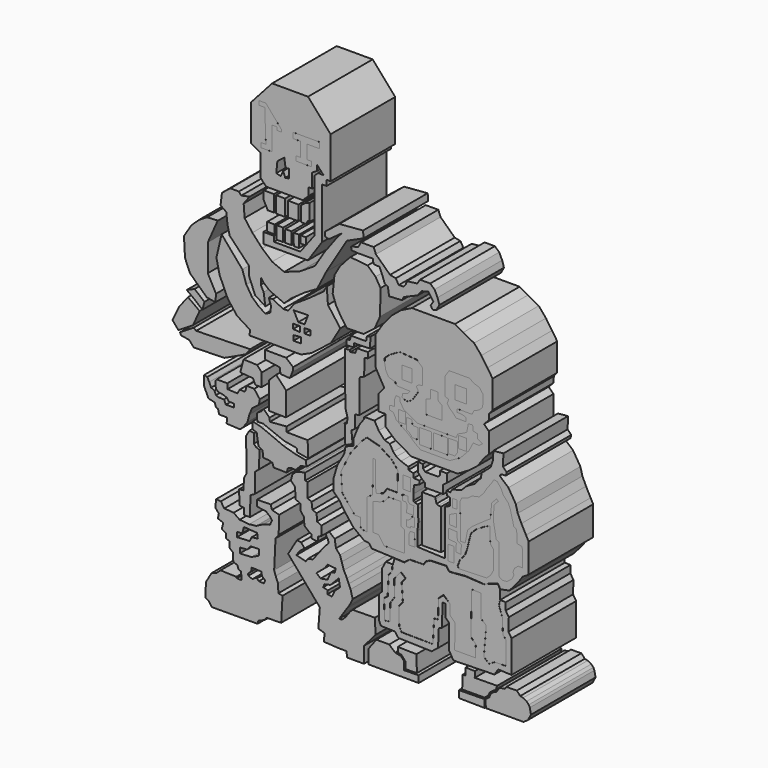
from build123d import *

# Parameters (mm, degrees)
F1_DEPTH      = 12.7
F1_DEPTH_BACK = 12.7
F0_W          = 2.3451782763
F0_H          = 2.7289353311
F3_DEPTH      = 12.7
F3_DEPTH_BACK = 12.7
F2_W          = 3.1842617318
F2_H          = 4.0236283094
F2_W_2        = 3.6299433559
F2_H_2        = 4.2267246172
F2_W_3        = 1.8677245826
F2_H_3        = 4.6415366232
F2_W_4        = 1.5032105148
F2_H_4        = 2.5777257979
F2_W_5        = 3.182772547
F2_H_5        = 4.0222080424
F2_W_6        = 3.6285351962
F2_H_6        = 4.2254780419
F2_W_7        = 2.2105854005
F2_H_7        = 3.4294971265
F2_W_8        = 1.8693469465
F2_H_8        = 4.6432167292
F2_W_9        = 1.5042312443
F2_H_9        = 2.5786831975
F2_W_10       = 3.7808120251
F2_H_10       = 4.7481860965
F2_W_11       = 4.3708886951
F2_H_11       = 4.6935402788
F2_W_12       = 2.4654623121
F2_H_12       = 3.6471767817
F2_W_13       = 2.2135460749
F2_H_13       = 3.4322766587
F2_W_14       = 3.7859473377
F2_H_14       = 4.7525740229
F2_W_15       = 4.3766628951
F2_H_15       = 4.6988725662
F2_W_16       = 2.4702642113
F2_H_16       = 3.651695326


# Not quite as in the source:
# - a feature names something its author has since deleted; it is built from what else it names


with BuildPart() as f1:
    # F0 (on Front) → F1 (new body, two sides)
    with BuildSketch(Plane.XZ) as f1_sk:
        Polygon((-9.5938611776, 66.9106543064), (-16.6862662882, 74.9939456582), (-27.994306758, 74.9939456582), (-34.6385799348, 67.5830319524), (-34.6385799348, 56.2110990286), (-31.6603220999, 54.5591711998), (-31.6603220999, 47.6847961545), (-29.7909770161, 45.815449208), (-18.3336883783, 45.815449208), (-16.5246427059, 47.5641936064), (-16.5246427059, 49.9762557447), (-15.3789138421, 49.9762557447), (-15.3789138421, 54.4385686517), (-13.9103056863, 55.3104877472), (-13.9103056863, 57.1270510554), (-11.8339713663, 54.8590533435), (-13.5205361214, 54.8850011104), (-14.5949935541, 53.9049506187), (-14.5949935541, 37.3129360378), (-17.3938885863, 33.6037576199), (-19.1130582243, 31.3254632056), (-27.4183992296, 31.3254632056), (-27.4183992296, 32.9865328968), (-30.7405348867, 32.9865328968), (-30.7405348867, 29.6643972397), (-16.7492311448, 29.6643972397), (-12.3410113156, 36.1170060933), (-12.3410113156, 52.1527044475), (-10.8716050163, 52.1527044475), (-10.8716050163, 53.877659142), (-9.5938611776, 53.877659142), align=None)
        Polygon((-26.3316370547, 54.0427602828), (-24.165680632, 55.7010732591), (-23.7595625222, 52.9597811401), (-22.728053189, 53.1125976231), (-22.728053189, 50.3538660705), (-23.861091584, 50.2184927464), (-24.5041102171, 51.8768019974), (-25.3163445741, 50.184648484), (-26.6700685024, 50.5569241941), align=None, mode=Mode.SUBTRACT)
        Polygon((-31.4840041101, 57.4934072793), (-29.9422182143, 57.4934072793), (-30.3007718176, 67.6046609879), (-32.0935472846, 67.6046609879), (-32.0935472846, 68.8936337829), (-29.9574602395, 68.8936337829), (-24.9686259777, 63.0946457386), (-24.9686259777, 62.4657310545), (-26.4403745532, 62.4657310545), (-26.5174116939, 63.4554550052), (-28.077730909, 63.4554550052), (-28.077730909, 56.0591891408), (-31.4840041101, 56.0591891408), align=None, mode=Mode.SUBTRACT)
        Polygon((-21.3707555085, 61.8773698807), (-21.3707555085, 63.4141266346), (-21.3707555085, 63.6133402586), (-13.1177809089, 63.6133402586), (-13.1177809089, 61.763536185), (-16.9881414622, 61.763536185), (-16.9881414622, 57.4662983418), (-15.6221324578, 57.4662983418), (-15.6221324578, 55.9295378625), (-20.4316228628, 55.9295378625), (-20.4316228628, 57.4093796313), (-19.0371554345, 57.4093796313), (-19.0371554345, 61.8773698807), align=None, mode=Mode.SUBTRACT)
    extrude(amount=F1_DEPTH)
    extrude(f1_sk.sketch, amount=-F1_DEPTH_BACK)


with BuildPart() as f1b:
    # F0 (on Front) → F1, piece 2 (new body, two sides)
    with BuildSketch(Plane.XZ) as f1_2_sk:
        Polygon((-30.6372623891, 44.5467084646), (-30.6372623891, 44.2908704281), (-30.6372623891, 41.903052479), (-29.358074069, 39.4299551845), (-27.3966528475, 39.4299551845), (-27.3966528475, 44.5467084646), align=None)
    extrude(amount=F1_DEPTH)
    extrude(f1_2_sk.sketch, amount=-F1_DEPTH_BACK)


with BuildPart() as f1c:
    # F0 (on Front) → F1, piece 3 (new body, two sides)
    with BuildSketch(Plane.XZ) as f1_3_sk:
        Polygon((-23.9142030478, 44.4402880967), (-26.7252419144, 44.472232461), (-26.7252419144, 39.3612533808), (-23.9142030478, 39.3612533808), align=None)
    extrude(amount=F1_DEPTH)
    extrude(f1_3_sk.sketch, amount=-F1_DEPTH_BACK)


with BuildPart() as f1d:
    # F0 (on Front) → F1, piece 4 (new body, two sides)
    with BuildSketch(Plane.XZ) as f1_4_sk:
        Polygon((-19.6976456791, 44.1527962685), (-22.9558944702, 44.1847406328), (-22.9558944702, 39.5529158413), (-19.6976456791, 39.5529158413), align=None)
    extrude(amount=F1_DEPTH)
    extrude(f1_4_sk.sketch, amount=-F1_DEPTH_BACK)


with BuildPart() as f1e:
    # F0 (on Front) → F1, piece 5 (new body, two sides)
    with BuildSketch(Plane.XZ) as f1_5_sk:
        Polygon((-17.4935366958, 45.2708229423), (-18.8671126962, 44.2805700004), (-18.8671126962, 39.5529158413), (-17.1741005033, 39.5529158413), (-16.8227199465, 40.5431687832), (-16.1519050598, 40.5431687832), (-16.1519050598, 45.7819215953), align=None)
    extrude(amount=F1_DEPTH)
    extrude(f1_5_sk.sketch, amount=-F1_DEPTH_BACK)


with BuildPart() as f1f:
    # F0 (on Front) → F1, piece 6 (new body, two sides)
    with BuildSketch(Plane.XZ) as f1_6_sk:
        Polygon((-19.0333388746, 33.6037576199), (-17.3938885863, 33.6037576199), (-17.3938885863, 35.8636565506), (-19.0333388746, 35.8636565506), (-19.0333388746, 35.5651788414), align=None)
    extrude(amount=F1_DEPTH)
    extrude(f1_6_sk.sketch, amount=-F1_DEPTH_BACK)


with BuildPart() as f1g:
    # F0 (on Front) → F1, piece 7 (new body, two sides)
    with BuildSketch(Plane.XZ) as f1_7_sk:
        Polygon((-21.2505981326, 35.8636565506), (-21.1653206497, 32.1540087461), (-19.5450149477, 32.1540087461), (-19.5450149477, 35.8636565506), align=None)
    extrude(amount=F1_DEPTH)
    extrude(f1_7_sk.sketch, amount=-F1_DEPTH_BACK)


with BuildPart() as f1h:
    # F0 (on Front) → F1, piece 8 (new body, two sides)
    with BuildSketch(Plane.XZ) as f1_8_sk:
        Polygon((-23.8516163081, 36.0342152417), (-23.8942559808, 32.1966484189), (-21.8475535512, 32.1966484189), (-21.8475535512, 36.0342152417), align=None)
    extrude(amount=F1_DEPTH)
    extrude(f1_8_sk.sketch, amount=-F1_DEPTH_BACK)


with BuildPart() as f1i:
    # F0 (on Front) → F1, piece 9 (new body, two sides)
    with BuildSketch(Plane.XZ) as f1_9_sk:
        Polygon((-26.5379119664, 36.2047739327), (-26.623191312, 32.1966484189), (-24.5338492095, 32.1966484189), (-24.5338492095, 36.2047739327), align=None)
    extrude(amount=F1_DEPTH)
    extrude(f1_9_sk.sketch, amount=-F1_DEPTH_BACK)


with BuildPart() as f1j:
    # F0 (on Front) → F1, piece 10 (new body, two sides)
    with BuildSketch(Plane.XZ) as f1_10_sk:
        with Locations((-28.3500943333, 34.8403062671)):
            Rectangle(F0_W, F0_H)
    extrude(amount=F1_DEPTH)
    extrude(f1_10_sk.sketch, amount=-F1_DEPTH_BACK)


with BuildPart() as f1k:
    # F0 (on Front) → F1, piece 11 (new body, two sides)
    with BuildSketch(Plane.XZ) as f1_11_sk:
        Polygon((-36.9369212724, 38.8479313689), (-35.0333526731, 41.3705967367), (-37.6954227686, 40.775667876), (-38.418225944, 41.6791699827), (-41.128732264, 41.6791699827), (-43.7488853931, 39.6011136472), (-44.2006364465, 35.9871052206), (-42.3936359584, 34.7222052515), (-42.0322343707, 31.4695984125), (-41.3094311953, 28.488041833), (-35.2559685707, 22.1635270864), (-35.2559685707, 19.3626713008), (-33.3586148918, 14.6644618362), (-30.1060080528, 12.5864073634), (-30.6481085718, 16.3811147213), (-31.5516106784, 18.097769469), (-31.42894949, 20.0820728757), (-30.6238532066, 18.9463123679), (-28.6898408085, 17.3346363008), (-24.1771470755, 15.4006257653), (-21.9745226204, 17.4420811236), (-17.7304428071, 20.4505436122), (-13.8624189422, 22.7068904787), (-10.961400345, 28.4014809877), (-4.491341766, 39.0913411975), (0.7715018001, 41.4606525215), (0.5989942583, 43.5738749802), (-6.8465704098, 42.9660752416), (-11.3291051239, 39.3952429295), (-11.3291051239, 38.0276888609), (-10.1135037839, 37.7237871289), (-6.0868188739, 40.610846132), (-7.7582728118, 38.7114658952), (-11.4810559899, 33.6971059442), (-14.5200621337, 28.8346949965), (-19.1545449197, 25.8716642857), (-24.1689067334, 24.0482613444), (-27.9676634818, 25.6437398493), (-31.0826450586, 28.3028688282), (-34.1976247728, 31.6457748413), (-36.6288311779, 34.9127091467), align=None)
    extrude(amount=F1_DEPTH)
    extrude(f1_11_sk.sketch, amount=-F1_DEPTH_BACK)


with BuildPart() as f1l:
    # F0 (on Front) → F1, piece 12 (new body, two sides)
    with BuildSketch(Plane.XZ) as f1_12_sk:
        Polygon((-0.9377481183, 38.5080315173), (-3.0890780035, 37.9343405366), (-3.1607891433, 37.7909205854), (-2.9456561897, 36.9303897023), (-1.2245918624, 36.7869660258), (3.723466536, 36.7869660258), (3.8668890484, 35.3527478874), (5.8030853979, 35.2093242109), (6.663617678, 33.2014150918), (7.3807276785, 31.1935078353), (8.3846813068, 30.6198205799), (8.8149476796, 28.0382242054), (12.8307631239, 28.2533578575), (13.4044513106, 29.3290223926), (15.0538031012, 30.0461333245), (17.7788212895, 31.1935078353), (18.9979076385, 32.7711515129), (21.1492385715, 33.3448387682), (22.7268803865, 31.0500860214), (21.8663476408, 29.8309996724), (22.4400348961, 28.7553351372), (23.6591231078, 29.0421787649), (24.5913658291, 30.7632423937), (24.0176785737, 32.6277278364), (23.0854358524, 34.5639251173), (21.7229258269, 35.7830114663), (18.4959303588, 35.7830114663), (17.6354013383, 34.4205051661), (14.4084058702, 34.0619497001), (13.978138566, 32.9145714641), (13.4044513106, 32.1974642575), (11.8268085644, 32.1257524192), (10.894565843, 33.7033942342), (9.1017913073, 34.0619497001), (4.6557090245, 38.2928960025), (3.938599024, 40.0856733322), (0, 40.0856733322), align=None)
    extrude(amount=F1_DEPTH)
    extrude(f1_12_sk.sketch, amount=-F1_DEPTH_BACK)


with BuildPart() as f1m:
    # F0 (on Front) → F1, piece 13 (new body, two sides)
    with BuildSketch(Plane.XZ) as f1_13_sk:
        Polygon((2.0290226676, 34.3684926629), (-3.3819169391, 34.9032784963), (-5.0103398971, 33.2014150918), (-6.7701800726, 31.1195589602), (-8.394648321, 28.276739642), (-8.936136961, 22.9972191155), (-7.8531587496, 20.0190264732), (-6.0933185741, 17.1085204929), (-4.4688507915, 14.8748783395), (0.8106696187, 15.0102507323), (4.1949781589, 17.5823252648), (5.9548197314, 21.508121863), (6.0901925899, 29.4274035841), (4.5334086753, 32.0671647787), align=None)
    extrude(amount=F1_DEPTH)
    extrude(f1_13_sk.sketch, amount=-F1_DEPTH_BACK)


with BuildPart() as f1n:
    # F0 (on Front) → F1, piece 14 (new body, two sides)
    with BuildSketch(Plane.XZ) as f1_14_sk:
        Polygon((-37.35839203, 20.4856079072), (-43.8636057079, 28.0750244856), (-45.4980805516, 21.0728552192), (-44.4747321308, 16.553055495), (-41.9163554907, 10.8393486589), (-39.0168614686, 7.087062113), (-34.9234566092, 4.5286854729), (-35.0940153003, 2.908379538), (-18.8909620047, 2.908379538), (-15.6503524631, 4.3581272475), (-9.5305331051, 9.1014830396), (-6.5489741974, 14.1610940918), (-10.4340352118, 19.4014050066), (-10.7954340056, 24.3706665933), (-11.7892883718, 22.6540118456), (-16.6681967676, 19.1303547472), (-20.8243075758, 16.4198484272), (-22.9927096516, 13.7093439698), (-24.5286636055, 13.7093439698), (-27.7812685817, 15.335646458), (-29.0461741388, 15.335646458), (-28.323372826, 13.2575919852), (-28.5944230855, 11.2698879093), (-30.1303770393, 10.5470865965), (-32.2987772524, 11.9926892221), (-34.2864841223, 13.7996925041), (-36.0934883356, 16.6908986866), align=None)
        Polygon((-21.2671738118, 5.9554395266), (-21.2671738118, 7.5206770562), (-18.9672354609, 7.7123385854), (-18.9672354609, 5.9554395266), align=None, mode=Mode.SUBTRACT)
        Polygon((-21.3949494064, 9.1498009861), (-21.3949494064, 10.6511516497), (-19.1588960588, 10.6511516497), (-19.1588960588, 8.9900828898), align=None, mode=Mode.SUBTRACT)
        Polygon((-19.7437535971, 11.6068609059), (-20.9376644343, 13.9094004408), (-21.1935024709, 14.4210755825), (-16.6737027466, 14.506354928), (-17.7823323756, 11.6068609059), align=None, mode=Mode.SUBTRACT)
        Polygon((-17.8172644228, 9.0539706871), (-17.8172644228, 10.5872638524), (-15.9006472677, 10.6511516497), (-15.9006472677, 9.0539706871), align=None, mode=Mode.SUBTRACT)
    extrude(amount=F1_DEPTH)
    extrude(f1_14_sk.sketch, amount=-F1_DEPTH_BACK)


with BuildPart() as f1o:
    # F0 (on Front) → F1, piece 15 (new body, two sides)
    with BuildSketch(Plane.XZ) as f1_15_sk:
        Polygon((-48.2119210064, 24.4022365659), (-45.1531931758, 31.3246250153), (-44.9922047555, 31.4856097102), (-48.4028458595, 31.2973856926), (-50.9676299989, 29.741641134), (-53.3509030938, 27.4967011064), (-55.6977577507, 23.7582940608), (-55.3757883608, 17.8018212318), (-53.8464225829, 14.0991490334), (-50.7876947522, 11.2014058977), (-48.5338903964, 9.1085908934), (-45.7971356809, 8.6256340146), (-45.636150986, 11.0404202715), (-48.2119210064, 15.8699918538), align=None)
    extrude(amount=F1_DEPTH)
    extrude(f1_15_sk.sketch, amount=-F1_DEPTH_BACK)


with BuildPart() as f1p:
    # F0 (on Front) → F1, piece 16 (new body, two sides)
    with BuildSketch(Plane.XZ) as f1_16_sk:
        Polygon((-52.33906582, 10.1660164073), (-54.8434145749, 9.0845925733), (-52.5667332113, 7.4339979328), (-49.8916320503, 5.2142329514), (-49.2655448616, 7.6047494076), align=None)
    extrude(amount=F1_DEPTH)
    extrude(f1_16_sk.sketch, amount=-F1_DEPTH_BACK)


with BuildPart() as f1q:
    # F0 (on Front) → F1, piece 17 (new body, two sides)
    with BuildSketch(Plane.XZ) as f1_17_sk:
        Polygon((-50.790656358, 4.5965607278), (-54.4437915087, 7.2289654054), (-57.129919529, 3.7907224614), (-59.3325421214, -0.6682488602), (-57.4522539973, -2.8708733153), (-52.8321154416, 0), align=None)
    extrude(amount=F1_DEPTH)
    extrude(f1_17_sk.sketch, amount=-F1_DEPTH_BACK)


with BuildPart() as f1r:
    # F0 (on Front) → F1, piece 18 (new body, two sides)
    with BuildSketch(Plane.XZ) as f1_18_sk:
        Polygon((-52.617225796, -0.6145262741), (-56.9150298834, -3.3006537706), (-56.6464141011, -4.0527693927), (-54.0677346289, -4.4825496152), (-52.617225796, -6.094226148), (-43.0546104908, -5.8793355711), (-39.5626462996, -4.267659504), (-36.2318493426, -2.655983204), (-34.8887853324, -0.8294165018), (-51.8651083112, -1.2591967825), align=None)
    extrude(amount=F1_DEPTH)
    extrude(f1_18_sk.sketch, amount=-F1_DEPTH_BACK)


with BuildPart() as f1s:
    # F0 (on Front) → F1, piece 19 (new body, two sides)
    with BuildSketch(Plane.XZ) as f1_19_sk:
        Polygon((-23.6031040549, 0.4885619273), (-30.1950573921, 0.5392691819), (-30.1950573921, -2.1482193843), (-25.5299843848, -2.8074146248), (-25.3778602928, -4.5821708627), (-22.4875435233, -4.7850008123), (-21.524105221, -2.7567071375), (-21.3719829917, -1.3876094017), align=None)
    extrude(amount=F1_DEPTH)
    extrude(f1_19_sk.sketch, amount=-F1_DEPTH_BACK)


with BuildPart() as f1t:
    # F0 (on Front) → F1, piece 20 (new body, two sides)
    with BuildSketch(Plane.XZ) as f1_20_sk:
        Polygon((-36.8002168834, -4.3107029051), (-36.9612015784, -4.3107029051), (-38.0076095462, -8.2548540086), (-33.9829660952, -8.5768252611), (-33.2585312426, -10.1866824552), (-31.3267037272, -10.1866824552), (-31.2462095171, -6.0815461911), (-32.695081085, -4.4716885313), align=None)
    extrude(amount=F1_DEPTH)
    extrude(f1_20_sk.sketch, amount=-F1_DEPTH_BACK)


with BuildPart() as f1u:
    # F0 (on Front) → F1, piece 21 (new body, two sides)
    with BuildSketch(Plane.XZ) as f1_21_sk:
        Polygon((-28.9138779044, -7.434383966), (-29.0096011013, -7.434383966), (-29.0096011013, -15.9537047148), (-23.6491281539, -16.049426049), (-23.5534086823, -8.5830567405), (-26.7122555524, -5.2327625453), align=None)
    extrude(amount=F1_DEPTH)
    extrude(f1_21_sk.sketch, amount=-F1_DEPTH_BACK)


with BuildPart() as f1v:
    # F0 (on Front) → F1, piece 22 (new body, two sides)
    with BuildSketch(Plane.XZ) as f1_22_sk:
        Polygon((-5.1528443582, -11.6437776014), (-4.9752146006, -17.6448337734), (-2.6907407378, -16.5448998462), (-3.0455661472, -12.9111642018), (-1.8998369342, -12.1272439137), (-1.929987804, -8.1473439932), (-0.5732035497, -7.9362886027), (-0.42929349, 2.6036400814), (0.9762255359, 3.2425122336), (0.9992049308, 8.3681419492), (2.2052354179, 8.7299505249), (2.0846324041, 10.4183927178), (-1.2922529131, 10.3580914438), (-1.8349663587, 8.9108552784), (-3.40280612, 8.6394986138), (-3.5535597708, 9.21236258), (-5.0912485458, 8.9711565524), (-4.961182829, -7.0438971743), (-4.7858525068, -7.9941847362), (-4.2383526452, -9.9451867864), (-4.5139719732, -11.4521170035), align=None)
    extrude(amount=F1_DEPTH)
    extrude(f1_22_sk.sketch, amount=-F1_DEPTH_BACK)


with BuildPart() as f1w:
    # F0 (on Front) → F1, piece 23 (new body, two sides)
    with BuildSketch(Plane.XZ) as f1_23_sk:
        Polygon((-3.4961928613, 11.9555769488), (-4.6345340088, 11.6994502023), (-4.6345340088, 10.1626897231), (-2.32939329, 10.2765234187), (-2.2155591287, 11.4717818797), (2.7931416407, 11.6140749305), (2.9354346916, 14.9437226355), (1.7970931949, 14.6591365337), (1.5694251051, 13.2362106815), (-3.2685245387, 13.2362106815), align=None)
    extrude(amount=F1_DEPTH)
    extrude(f1_23_sk.sketch, amount=-F1_DEPTH_BACK)


with BuildPart() as f1x:
    # F0 (on Front) → F1, piece 24 (new body, two sides)
    with BuildSketch(Plane.XZ) as f1_24_sk:
        Polygon((-32.6734371483, -17.6987983286), (-32.6734371483, -19.6284465492), (-32.5862728059, -20.1711598784), (-30.7437889278, -20.1108586043), (-28.5126324743, -21.0153814405), (-24.2312233895, -22.7038245648), (-20.2513244003, -23.4274435788), (-20.1307218522, -24.5128702372), (-16.6332330555, -25.1158848405), (-16.8141368777, -20.1108586043), (-23.4473049641, -20.0505573303), (-23.4473049641, -18.4827186167), (-28.6935362965, -18.9048293978), (-28.8141407073, -17.8194008768), (-30.6231863797, -16.0103552043), (-31.3468053937, -16.8545767665), align=None)
    extrude(amount=F1_DEPTH)
    extrude(f1_24_sk.sketch, amount=-F1_DEPTH_BACK)


with BuildPart() as f1y:
    # F0 (on Front) → F1, piece 25 (new body, two sides)
    with BuildSketch(Plane.XZ) as f1_25_sk:
        Polygon((-31.2966257334, -21.257204935), (-34.0757220984, -20.5111056566), (-34.0757220984, -22.7471590042), (-32.8299216926, -23.1943689287), (-32.2868786752, -26.7720539123), (-30.9771914035, -27.6025887579), (-30.7855289429, -29.5192059129), (-28.9008561522, -29.6469796449), (-27.8467163444, -29.9983602017), (-27.5272801518, -31.1802737415), (-23.4384965152, -31.2441606075), (-23.023230955, -29.9025289714), (-21.7774286866, -29.4872615486), (-20.5955151469, -29.5830927789), (-19.7330377996, -28.6886710674), (-18.9983341843, -27.9220249504), (-17.1775482595, -27.6025887579), (-17.3692107201, -25.8776322007), (-20.946893841, -25.1543261111), (-24.3968050927, -24.1640750319), (-27.3995064199, -22.8863302618), align=None)
    extrude(amount=F1_DEPTH)
    extrude(f1_25_sk.sketch, amount=-F1_DEPTH_BACK)


with BuildPart() as f1z:
    # F0 (on Front) → F1, piece 26 (new body, two sides)
    with BuildSketch(Plane.XZ) as f1_26_sk:
        Polygon((-43.0968850851, -17.3945352435), (-44.8567271233, -17.3945352435), (-45.6112548709, -17.0357543975), (-46.1307689548, -15.951551497), (-47.1697971225, -15.4546266422), (-47.7570705116, -14.0993734822), (-48.344347626, -12.8796454519), (-49.3616610765, -12.6537699252), (-49.3616610765, -15.761744231), (-47.9702912271, -18.7482573092), (-45.9973849356, -19.1603135318), (-45.6689596176, -20.3727260232), (-44.9827052653, -20.6235628575), (-44.6536689997, -22.0648795366), (-42.1492792666, -22.0648795366), (-42.2846525908, -23.8247197121), (-38.0881093442, -24.0277796984), (-37.2081883252, -23.2832320035), (-35.7190929353, -21.2526451796), (-35.1099185646, -18.9513172954), (-34.2976860702, -16.9884171337), (-32.1317277849, -15.2962636203), (-31.8609811366, -13.6717958376), (-33.6208231747, -11.3704660907), (-35.9221510589, -11.3027794287), (-36.531329155, -13.1303062662), (-38.155797869, -13.0626205355), (-38.9003455639, -14.3486568704), (-42.0139059424, -14.2132854089), (-42.0815944672, -12.5888166949), (-45.3982166946, -12.5888166949), (-45.7513257861, -13.1409596652), (-45.6944070756, -15.1330558583), (-44.9921004474, -15.9054398537), (-43.3676317334, -16.1761846393), (-42.2846525908, -16.5823008865), (-41.6077896953, -17.4622200429), (-39.9833209813, -17.529906705), (-39.9156361818, -18.6128858477), (-42.5553955138, -18.6805725098), align=None)
    extrude(amount=F1_DEPTH)
    extrude(f1_26_sk.sketch, amount=-F1_DEPTH_BACK)


with BuildPart() as f1ba:
    # F0 (on Front) → F1, piece 27 (new body, two sides)
    with BuildSketch(Plane.XZ) as f1_27_sk:
        Polygon((-33.6043462157, -23.650649935), (-35.135909915, -23.435274139), (-36.1285246909, -25.1578874886), (-36.0905379057, -35.6804467738), (-36.8502885103, -37.1619611979), (-36.9642525911, -40.580842644), (-38.3318029344, -40.6948067248), (-38.2938161492, -45.1773405075), (-36.8882752955, -45.3292913735), (-36.8123017251, -47.3046451807), (-34.9509119987, -47.3426319659), (-34.7989611328, -41.1886461079), (-33.4396325052, -40.4247939587), (-33.4396325052, -34.3261547387), (-32.0843793452, -33.1516042352), (-31.9770611823, -27.7427956462), (-33.0539382994, -27.3120421916), (-33.7239988148, -26.6180541366), align=None)
    extrude(amount=F1_DEPTH)
    extrude(f1_27_sk.sketch, amount=-F1_DEPTH_BACK)


with BuildPart() as f1bb:
    # F0 (on Front) → F1, piece 28 (new body, two sides)
    with BuildSketch(Plane.XZ) as f1_28_sk:
        Polygon((-18.8277959824, -29.6179540455), (-20.5805432051, -30.192617327), (-21.6056704521, -31.1802737415), (-22.0880825073, -33.0267883837), (-20.76144889, -34.3534238636), (-20.6408444792, -37.7303063869), (-19.0127044916, -38.3936241269), (-19.0730057657, -40.3232723475), (-17.9272778332, -41.8308116496), (-17.860205844, -44.0748855472), (-16.3803622127, -45.3839786351), (-15.6404413283, -45.7823984325), (-15.5835244805, -46.9207391143), (-13.6483442038, -47.1484065056), (-13.5345105082, -45.7823984325), (-12.3961688951, -45.1563112438), (-12.510003522, -42.3673763871), (-13.8760125265, -41.6843704879), (-13.9898471534, -39.4076891243), (-15.29893931, -38.9523506165), (-15.5835244805, -36.7895029485), (-16.8357007205, -36.2203344703), (-16.8357007205, -31.7238867283), (-17.5756216049, -31.5531343222), (-17.6325384527, -29.3902866542), align=None)
    extrude(amount=F1_DEPTH)
    extrude(f1_28_sk.sketch, amount=-F1_DEPTH_BACK)


with BuildPart() as f1bc:
    # F0 (on Front) → F1, piece 29 (new body, two sides)
    with BuildSketch(Plane.XZ) as f1_29_sk:
        Polygon((-28.4168235958, -41.6801795363), (-32.7146276832, -41.7402908206), (-32.7146276832, -43.6743050814), (-29.9210548401, -44.0503619611), (-28.631715104, -45.1248139143), (-28.040766716, -45.9843724966), (-28.631715104, -47.3811589181), (-30.6731704623, -47.9183867574), (-32.9832397401, -49.100279808), (-35.1858660579, -49.3688955903), (-38.1943285465, -49.100279808), (-40.0746166706, -47.7572157979), (-43.0293567479, -47.5423261523), (-44.103808701, -45.9306500852), (-45.6080399454, -45.8232052624), (-45.8229295909, -48.2407212257), (-44.7484776378, -49.5300628245), (-45.0170896947, -50.9805716574), (-43.3516912162, -51.6252405941), (-43.7814742327, -53.4518063068), (-42.4921326339, -54.2039237916), (-42.4921326339, -55.6007102132), (-41.4176806808, -56.0842119157), (-41.3639582694, -57.9107776284), (-40.3432287276, -58.770339936), (-40.1820614934, -61.2953007221), (-38.8927198946, -61.9399696589), (-38.5166630149, -63.0144178867), (-37.7645455301, -63.2293075323), (-37.5496558845, -65.6468272209), (-39.0538871288, -65.5931010842), (-39.215054363, -65.2170479298), (-44.2112535238, -65.0558769703), (-45.5005951226, -66.237770021), (-47.0048263669, -66.7212754488), (-48.7776696682, -69.7233527899), (-48.9925593138, -74.1285979748), (-47.9181073606, -74.7732669115), (-46.8973815441, -76.1163309216), (-32.553460449, -76.0626122355), (-32.284848392, -75.0418826938), (-31.3178412616, -74.7195482254), (-30.2433911711, -74.2360427976), (-29.8136100173, -73.483929038), (-25.1397490501, -73.3764842153), (-24.7099678963, -65.7478794456), (-25.9993094951, -65.4792711139), (-26.1604785919, -62.7394169569), (-26.85886994, -60.9665736556), (-27.3423735052, -59.5160648227), (-26.9125942141, -50.5981221795), (-25.9455870837, -49.3087805808), (-25.7306974381, -43.6679162085), (-28.040766716, -43.0769659579), align=None)
        Polygon((-34.1644622386, -64.2259716988), (-35.4741513729, -63.714876771), (-35.5060957372, -63.0760043859), (-34.579731524, -62.2454695404), (-34.451957792, -61.0954985023), (-31.3534252346, -61.2232722342), (-31.1937071383, -62.3732432723), (-30.1395691931, -63.3315518498), (-30.5548347533, -64.2259716988), (-32.1839600801, -64.1620829701), (-32.7589437366, -63.5870993137), (-33.2380980253, -63.5870993137), align=None, mode=Mode.SUBTRACT)
        Polygon((-38.1465218961, -58.3931319416), (-38.1465218961, -56.7442439497), (-35.8651801944, -56.5861277282), (-34.8487384617, -55.3438141942), (-32.1156457067, -55.2308782935), (-32.0478826761, -57.0378787816), (-34.487336874, -58.2124330103), align=None, mode=Mode.SUBTRACT)
        Polygon((-39.0662886202, -54.2039237916), (-39.0662886202, -52.7116432786), (-37.3587757349, -52.5978058577), (-36.8465222418, -50.6626293063), (-32.6915755868, -50.9472116828), (-32.4639081955, -52.483972162), (-34.3990884721, -52.7116432786), (-35.0251756608, -53.963817656), align=None, mode=Mode.SUBTRACT)
    extrude(amount=F1_DEPTH)
    extrude(f1_29_sk.sketch, amount=-F1_DEPTH_BACK)


with BuildPart() as f1bd:
    # F0 (on Front) → F1, piece 30 (new body, two sides)
    with BuildSketch(Plane.XZ) as f1_30_sk:
        Polygon((-19.426131621, -51.6865924001), (-17.7577332582, -50.3934485057), (-18.8531130552, -49.0724369884), (-20.1647710055, -48.8816089928), (-22.9407288134, -53.5720214248), (-12.9855694249, -65.1544630527), (-13.4641826153, -71.1849927902), (-11.5497289225, -71.7593356967), (-11.6454521194, -74.2481201887), (-6.9550401531, -74.5352879167), (-4.6576941386, -74.5352879167), (-4.3705268763, -76.2583017349), (0.8942213608, -76.2583017349), (0.8942206623, -71.2807178497), (4.5316843316, -67.0689195395), (4.3402379379, -62.3785071075), (-2.7432409115, -62.474232167), (-3.6047447938, -63.4314566851), (-4.8491400667, -65.1544705033), (-5.9978123754, -66.3031414151), (-6.8593169563, -66.3031414151), (-5.9183971025, -64.8603662848), (-4.3988940306, -62.581114471), (-3.7004679907, -61.6127252579), (-2.6475179475, -59.5068261027), (-3.3175775316, -57.0180378854), (-3.8919141516, -55.6779205799), (-4.4662486762, -54.3378032744), (-5.4234764539, -52.4233467877), (-6.0935355723, -50.3174476326), (-6.6678719595, -48.5944412649), (-7.9122660682, -47.1585988998), (-8.2951579243, -44.6698106825), (-10.0181661546, -43.2339683175), (-11.1668379977, -44.2869178951), (-10.4010561481, -45.6270352006), (-10.2167800069, -46.425241977), (-12.3155107722, -48.8816089928), (-15.1871917769, -52.6147931814), (-16.7187545449, -52.9019609094), (-17.3888131976, -53.8591891527), (-20.3562173992, -53.0934073031), align=None)
        Polygon((-10.4784592986, -59.6494115889), (-11.9485352188, -59.2550002038), (-11.518268846, -58.2510456443), (-9.6537834033, -57.8566379845), (-7.0363315754, -55.1674738526), (-6.6419215873, -57.6056502759), (-8.2195624709, -58.9681565762), (-9.1876611114, -60.9402097762), (-10.5860261247, -60.7250779867), align=None, mode=Mode.SUBTRACT)
        Polygon((-12.714728713, -57.0676513016), (-14.0428608283, -55.9809990227), (-13.1171932444, -55.1760718226), (-11.547582224, -53.8881830871), (-10.5414213613, -52.5198057294), (-7.9656485468, -52.7612827718), (-8.3278669044, -54.0894158185), (-9.4950133935, -54.2906485498), (-10.5414213613, -56.7054338753), align=None, mode=Mode.SUBTRACT)
    extrude(amount=F1_DEPTH)
    extrude(f1_30_sk.sketch, amount=-F1_DEPTH_BACK)


with BuildPart() as f1be:
    # F0 (on Front) → F1, piece 31 (new body, two sides)
    with BuildSketch(Plane.XZ) as f1_31_sk:
        Polygon((-29.9574602395, 68.8925981522), (-32.0922508836, 68.8925981522), (-32.0922508836, 67.6055178046), (-30.2996076643, 67.6055178046), (-29.939731583, 57.4920475483), (-31.483117491, 57.4920475483), (-31.483117491, 56.0601837933), (-28.0790179968, 56.0601837933), (-28.0956011266, 63.473932445), (-26.5090446919, 63.4602755308), (-26.436150074, 62.4692924321), (-24.9725058675, 62.4692924321), (-24.9725058675, 63.093483448), align=None)
    extrude(amount=F1_DEPTH)
    extrude(f1_31_sk.sketch, amount=-F1_DEPTH_BACK)


with BuildPart() as f1bf:
    # F0 (on Front) → F1, piece 32 (new body, two sides)
    with BuildSketch(Plane.XZ) as f1_32_sk:
        Polygon((-13.1213907152, 63.6110603809), (-21.3671550155, 63.6095330119), (-21.3671550155, 61.8804320693), (-19.0351754427, 61.8804320693), (-19.0351754427, 57.4064180255), (-20.4279664904, 57.4064180255), (-20.4279664904, 55.9322498739), (-15.6266130507, 55.9322498739), (-15.6266130507, 57.4618503451), (-16.9916376472, 57.4618503451), (-16.9916376472, 61.7666766047), (-13.1213907152, 61.7666766047), align=None)
    extrude(amount=F1_DEPTH)
    extrude(f1_32_sk.sketch, amount=-F1_DEPTH_BACK)


with BuildPart() as f3:
    # F2 (on Front) → F3 (new body, two sides)
    with BuildSketch(Plane.XZ) as f3_sk:
        Polygon((19.411213696, -14.8924924433), (17.8433749825, -14.8924924433), (17.8433749825, -17.7266635001), (18.9891029149, -19.0532971174), (20.0142282993, -19.8975186795), (20.0142282993, -21.2241522968), (25.8031748235, -21.2241522968), (25.8031748235, -18.5708850622), (26.948902756, -17.7266635001), (26.948902756, -15.0733962655), (24.7780475765, -15.0733962655), (24.7780475765, -16.4000298828), (24.1750329733, -16.8824419379), (20.1951339841, -16.8824419379), (19.411213696, -16.1588247865), align=None)
    extrude(amount=F3_DEPTH)
    extrude(f3_sk.sketch, amount=-F3_DEPTH_BACK)


with BuildPart() as f3b:
    # F2 (on Front) → F3, piece 2 (new body, two sides)
    with BuildSketch(Plane.XZ) as f3_2_sk:
        Polygon((23.2366155833, -22.8002108634), (19.1131997854, -22.8002108634), (19.1131997854, -37.5137813389), (25.1433514059, -37.5137813389), (25.1433514059, -24.9107647687), (24.2991298437, -24.8504634947), (23.6961152405, -24.5489552617), (23.3946070075, -23.2826229185), align=None)
    extrude(amount=F3_DEPTH)
    extrude(f3_2_sk.sketch, amount=-F3_DEPTH_BACK)


with BuildPart() as f3c:
    # F2 (on Front) → F3, piece 3 (new body, two sides)
    with BuildSketch(Plane.XZ) as f3_3_sk:
        Polygon((9.8529430106, -45.790258795), (7.7470429242, -45.790258795), (6.6309138201, -47.9049906135), (6.5706125461, -54.4175542891), (5.5454866961, -55.5029809475), (5.6057879701, -62.5582560897), (6.2045394443, -64.0260279179), (10.657816194, -64.1292333603), (11.696241796, -65.5733346939), (22.1887063235, -65.8748447895), (24.1786558181, -64.3070042133), (24.419862777, -58.6386583745), (25.3846868873, -58.3371520042), (25.6258919835, -51.2215718627), (26.6044139862, -51.2464530766), (26.5086907893, -55.0753623247), (27.6573635638, -56.2240332365), (27.6573635638, -63.8818517327), (28.9974808693, -66.1791935563), (41.9200435281, -65.8920258284), (43.0687181652, -64.0732944012), (47.2805164754, -64.2647370696), (47.2805164754, -54.1181340814), (46.3232882321, -52.5865703821), (46.4190095663, -48.5662184656), (45.4617850482, -47.0346547663), (45.4617850482, -44.7373092175), (43.7387749553, -44.6415878832), (43.3558858931, -46.2688729167), (44.4088354707, -49.2362752557), (44.6002818644, -54.0224127471), (45.5575101078, -55.0753623247), (45.5575101078, -62.3502843082), (42.0157685876, -62.4460093677), (40.1970371604, -63.4989589453), (38.5697484016, -62.0631165802), (39.3355339766, -53.160905838), (37.6125238836, -51.7250671983), (37.6125238836, -44.7373092175), (34.7408428788, -44.6415878832), (34.5494002104, -57.9470433295), (36.0809601843, -59.3828819692), (35.8895137906, -63.2117912173), (29.3803717941, -63.2117912173), (29.5718181878, -55.6496977806), (27.9445312917, -54.0224127471), (27.9445312917, -50.8635602891), (25.9343553334, -49.1405539215), (24.4027916342, -50.480671227), (24.2113471031, -56.4154796302), (22.9669511318, -56.6069222987), (22.584060207, -63.7861266732), (12.7246240154, -63.6904016137), (11.9588421658, -62.254562974), (11.8631189689, -56.7026473582), (13.1075140089, -55.1710836589), (12.7246240154, -49.8106107116), (13.969018124, -48.3747720718), (12.4374544248, -47.1303761005), (10.4272784665, -49.6191680431), (10.5230016634, -54.7881908715), (9.1828834265, -56.7026473582), (9.087161161, -61.967395246), (7.364152465, -62.1588379145), (7.1727074683, -56.0325868428), (8.3298254758, -55.1587231457), (8.6085479707, -49.1405539215), (9.6614966169, -47.8004366159), align=None)
    extrude(amount=F3_DEPTH)
    extrude(f3_3_sk.sketch, amount=-F3_DEPTH_BACK)


with BuildPart() as f3d:
    # F2 (on Front) → F3, piece 4 (new body, two sides)
    with BuildSketch(Plane.XZ) as f3_4_sk:
        Polygon((2.2517784964, -71.7037245631), (2.2517784964, -75.5369588733), (2.2456638981, -75.9565010667), (18.095811829, -75.9841650724), (18.031924963, -73.8758891821), (13.4540820119, -73.9403673525), (13.5598191991, -71.5120583773), (12.5376228243, -70.3620910645), (10.6848934665, -69.9787661433), (8.8321631774, -68.3176964521), (4.8072678037, -68.3176964521), align=None)
    extrude(amount=F3_DEPTH)
    extrude(f3_4_sk.sketch, amount=-F3_DEPTH_BACK)


with BuildPart() as f3e:
    # F2 (on Front) → F3, piece 5 (new body, two sides)
    with BuildSketch(Plane.XZ) as f3_5_sk:
        Polygon((11.509006843, -68.1123957038), (11.53915748, -68.3536008), (11.53915748, -69.68023628), (12.6245850697, -69.8912888765), (13.8909174129, -71.3083744049), (13.92106805, -73.4792277217), (17.5391584635, -73.4189301729), (17.3884052783, -68.2329982519), align=None)
    extrude(amount=F3_DEPTH)
    extrude(f3_5_sk.sketch, amount=-F3_DEPTH_BACK)


with BuildPart() as f3f:
    # F2 (on Front) → F3, piece 6 (new body, two sides)
    with BuildSketch(Plane.XZ) as f3_6_sk:
        Polygon((38.7321710587, -73.72418046), (30.7547785342, -73.8381445408), (30.7547785342, -76.0414227843), (38.808144629, -76.1553868651), align=None)
    extrude(amount=F3_DEPTH)
    extrude(f3_6_sk.sketch, amount=-F3_DEPTH_BACK)


with BuildPart() as f3g:
    # F2 (on Front) → F3, piece 7 (new body, two sides)
    with BuildSketch(Plane.XZ) as f3_7_sk:
        Polygon((35.7636064291, -66.9536069036), (32.8658632934, -66.8731182814), (32.8658632934, -69.1269189119), (31.8596996367, -69.2074075341), (31.7792072892, -73.3125433326), (38.8223342597, -73.2723027468), (39.8687422276, -72.427123785), (40.4724404216, -71.3002234697), (41.1968752742, -70.6965252757), (42.3237755895, -69.9720904231), (42.7664853632, -68.7244534492), (35.7233583927, -68.8049420714), align=None)
    extrude(amount=F3_DEPTH)
    extrude(f3_7_sk.sketch, amount=-F3_DEPTH_BACK)


with BuildPart() as f3h:
    # F2 (on Front) → F3, piece 8 (new body, two sides)
    with BuildSketch(Plane.XZ) as f3_8_sk:
        Polygon((40.251083672, -72.7893412113), (39.3052920699, -73.4936520457), (39.1395650804, -73.6936181784), (39.2027460039, -76.079569757), (51.0757006705, -76.0237947106), (52.4053946137, -75.092881918), (53.3972711746, -73.2598043978), (53.0112311244, -71.4450851083), (52.6883378625, -70.7233175635), (52.0235523582, -70.0205489993), (50.9029217064, -69.4317370653), (50.0102117658, -69.2038163543), (48.9275641739, -68.0451914668), (45.6606335938, -68.0831819773), (45.201394707, -68.7848255038), (43.5311682522, -69.0061748028), (42.5652526319, -70.4550519586), (41.6597090662, -70.8172693849), (40.7944098115, -71.5618282557), align=None)
    extrude(amount=F3_DEPTH)
    extrude(f3_8_sk.sketch, amount=-F3_DEPTH_BACK)


with BuildPart() as f3i:
    # F2 (on Front) → F3, piece 9 (new body, two sides)
    with BuildSketch(Plane.XZ) as f3_9_sk:
        Polygon((4.8100892454, -27.8926938772), (4.8788301647, -27.7793295681), (6.9559456266, -27.0710128224), (8.171393536, -25.3861583769), (11.4074870944, -25.4249107093), (11.5326540545, -19.3315073848), (9.6515780315, -16.9598422945), (5.6938042647, -14.4064399843), (1.7834793543, -13.359323144), (0.0197774447, -15.0459936151), (-3.1720004044, -19.0298762172), (-6.3057861459, -25.3135934472), (-5.9224626218, -31.1912186444), (-1.980755711, -36.0438488424), (-0.18749437, -36.0453985631), (-0.104695045, -39.1537784858), (1.8284186246, -39.4873106011), (1.8458900095, -39.4903250477), (1.8498733407, -29.7824908048), (3.6118254066, -28.6000333726), (3.7727496209, -18.4618160129), (3.7727496209, -18.448041752), (4.5599858277, -18.4956751764), (4.4624623843, -25.9686578065), align=None)
    extrude(amount=F3_DEPTH)
    extrude(f3_9_sk.sketch, amount=-F3_DEPTH_BACK)


with BuildPart() as f3j:
    # F2 (on Front) → F3, piece 10 (new body, two sides)
    with BuildSketch(Plane.XZ) as f3_10_sk:
        Polygon((12.5512035929, -27.5318897338), (8.7034376338, -27.6120528579), (7.410542873, -29.0550756119), (6.0419713729, -29.779612506), (3.7883551914, -30.3430166095), (3.7883551914, -38.9545334723), (5.4785431724, -39.0350180932), (7.2494158521, -41.53034091), (13.6876897886, -41.53034091), (13.6782713234, -35.0915119052), (12.4707330288, -34.2913835954), align=None)
    extrude(amount=F3_DEPTH)
    extrude(f3_10_sk.sketch, amount=-F3_DEPTH_BACK)


with BuildPart() as f3k:
    # F2 (on Front) → F3, piece 11 (new body, two sides)
    with BuildSketch(Plane.XZ) as f3_11_sk:
        Polygon((8.8738944357, 11.8528466412), (7.4505838566, 10.5184940621), (7.4110946494, 9.1180661693), (7.7724962372, 7.1755368263), (8.5851195088, 5.6405814991), (10.6631761153, 4.962954689), (11.2955628349, 4.0595442914), (15.4081759974, 3.8787701633), (14.6419124615, 2.9719617509), (13.0144953728, 2.4746954441), (12.8904338714, 1.4012731254), (14.2766190693, 0.730538289), (15.9806408657, 1.5377065266), (18.0044658619, 4.5734448358), (17.709183215, 5.3677497596), (17.2794390956, 5.8452422959), (18.0364142214, 6.5265212356), (19.2315187305, 6.7085986957), (19.2264536499, 11.7355822865), (17.5550207706, 13.286102042), (12.1082141995, 13.6946121137), align=None)
        with Locations((14.4296702929, 8.3201155066)):
            Rectangle(F2_W, F2_H, mode=Mode.SUBTRACT)
    extrude(amount=F3_DEPTH)
    extrude(f3_11_sk.sketch, amount=-F3_DEPTH_BACK)


with BuildPart() as f3l:
    # F2 (on Front) → F3, piece 12 (new body, two sides)
    with BuildSketch(Plane.XZ) as f3_12_sk:
        Polygon((26.3629853725, 11.6480914876), (26.365365833, 6.0368538834), (27.5196485555, 5.6154328279), (27.0641141025, 4.3627084233), (27.8609518347, 3.2243675087), (28.8273151964, 2.3148490643), (29.9091748893, 1.1760494672), (33.0383120829, 1.1760494672), (33.0383120829, 2.3133222744), (31.843919307, 2.7683301984), (30.1350746304, 2.8822531458), (30.1350746304, 3.8516142422), (34.9162829847, 3.8516142422), (35.4280397296, 5.0457133912), (37.0792179113, 5.7291732426), (38.2171032441, 6.8670590408), (38.3309369397, 10.5097498745), (37.1933562092, 12.0454853497), (35.3158600628, 12.6713173985), (34.1199375689, 13.5824959091), (27.6894114359, 13.5824959091), align=None)
        with Locations((31.2793934718, 8.2185673527)):
            Rectangle(F2_W_2, F2_H_2, mode=Mode.SUBTRACT)
    extrude(amount=F3_DEPTH)
    extrude(f3_12_sk.sketch, amount=-F3_DEPTH_BACK)


with BuildPart() as f3m:
    # F2 (on Front) → F3, piece 13 (new body, two sides)
    with BuildSketch(Plane.XZ) as f3_13_sk:
        Polygon((13.1141859401, -19.9630289751), (13.1142763421, -23.8833520561), (15.5840891304, -23.9370453584), (15.5840891304, -20.0167223811), align=None)
    extrude(amount=F3_DEPTH)
    extrude(f3_13_sk.sketch, amount=-F3_DEPTH_BACK)


with BuildPart() as f3n:
    # F2 (on Front) → F3, piece 14 (new body, two sides)
    with BuildSketch(Plane.XZ) as f3_14_sk:
        Polygon((14.6602072638, -25.3948126497), (12.9216276109, -25.4025906324), (12.9615227783, -26.0908916892), (12.9615227783, -27.1095056087), (14.028663747, -27.1934978664), (14.4094737044, -27.6758577675), (14.3080983809, -30.1088692563), (16.4102148265, -30.1088692563), (16.5622463779, -27.4229816162), (15.3675985136, -27.3553599609), (14.8375943041, -26.9659552723), align=None)
    extrude(amount=F3_DEPTH)
    extrude(f3_14_sk.sketch, amount=-F3_DEPTH_BACK)


with BuildPart() as f3o:
    # F2 (on Front) → F3, piece 15 (new body, two sides)
    with BuildSketch(Plane.XZ) as f3_15_sk:
        Polygon((16.7892678302, -33.40784089), (16.7178865522, -30.6571312249), (16.0966416589, -30.5854492649), (15.5697613955, -31.3995219767), (14.8279098794, -31.9738574326), (14.3259083852, -31.9733321667), (14.3259083852, -33.934533596), (15.4256401584, -33.934533596), (15.6650380421, -33.3839205131), align=None)
    extrude(amount=F3_DEPTH)
    extrude(f3_15_sk.sketch, amount=-F3_DEPTH_BACK)


with BuildPart() as f3p:
    # F2 (on Front) → F3, piece 16 (new body, two sides)
    with BuildSketch(Plane.XZ) as f3_16_sk:
        Polygon((16.8296981012, -34.8238106071), (15.4489697888, -34.8470285535), (15.1187284069, -35.6099568307), (15.1187284069, -38.7751497328), (16.8961550268, -38.7450258294), align=None)
    extrude(amount=F3_DEPTH)
    extrude(f3_16_sk.sketch, amount=-F3_DEPTH_BACK)


with BuildPart() as f3q:
    # F2 (on Front) → F3, piece 17 (new body, two sides)
    with BuildSketch(Plane.XZ) as f3_17_sk:
        Polygon((31.2190782279, -32.4576869607), (32.7085070312, -32.4576869607), (33.4891026329, -28.6585802484), (34.8305478692, -27.2532589734), (36.5037880838, -26.0431521094), (38.9426494261, -24.3269164189), (40.6593007876, -23.1975410134), (41.0206843709, -18.7706005004), (42.5120741129, -17.0532403005), (43.190511959, -17.4603033811), (41.7449093333, -19.1317815334), (41.6093881338, -23.558781931), (42.4676440858, -28.2565902607), (43.3259183306, -28.7986602634), (43.3259183306, -38.2617617486), (44.4757379591, -39.005861893), (45.8289057874, -38.8705443655), (47.3854927338, -37.720023255), (48.0620065594, -36.2993457107), (47.723487322, -35.6900133193), (48.1972920939, -34.4716608524), (49.3486436462, -33.4557635203), (50.7699615866, -33.5234440853), (50.7699545124, -31.6293654135), (50.7022704095, -28.9219454181), (50.6345855396, -27.7036605974), (49.009919777, -27.2974922939), (49.0776184019, -25.4018935374), (48.8069221518, -23.507032823), (47.9271845217, -22.8303099933), (47.6563972612, -21.4763643763), (47.2501628101, -19.9868213419), (46.9118766487, -18.4977259487), (46.1674309615, -16.873849381), (44.7459382598, -15.3846670386), (43.9337437101, -13.6249171477), (42.7831095029, -12.2035442199), (41.7685204465, -12.000625478), (40.8890770796, -13.4212635458), (39.738442176, -14.8426373337), (38.5877527297, -16.7378857732), (37.0983023483, -18.2950708768), (34.8647820062, -18.7688477497), (33.7146110833, -19.6483917534), (31.6158570349, -20.3259289265), (31.14243038, -21.4082319289), align=None)
    extrude(amount=F3_DEPTH)
    extrude(f3_17_sk.sketch, amount=-F3_DEPTH_BACK)


with BuildPart() as f3r:
    # F2 (on Front) → F3, piece 18 (new body, two sides)
    with BuildSketch(Plane.XZ) as f3_18_sk:
        Polygon((31.1442632228, -37.5814437866), (30.3554423153, -39.661064744), (30.8681465685, -40.2319021523), (39.4731179086, -39.947430113), (40.6916961074, -38.8005338609), (41.6239388287, -37.1511802077), (41.6239388287, -31.3425883651), (40.6200923026, -30.1239825785), (40.4551066458, -25.211956352), (38.7024033604, -26.0542214736), (36.2229248403, -27.5419056416), (34.5650438853, -29.1997865966), (34.0232923627, -31.1862584203), (33.4138981998, -33.7807610631), (32.6563119888, -35.9320901334), align=None)
    extrude(amount=F3_DEPTH)
    extrude(f3_18_sk.sketch, amount=-F3_DEPTH_BACK)


with BuildPart() as f3s:
    # F2 (on Front) → F3, piece 19 (new body, two sides)
    with BuildSketch(Plane.XZ) as f3_19_sk:
        Polygon((30.2514377981, -32.6221548021), (30.1311910152, -30.2106887102), (27.5394897877, -30.0901449), (27.5394897877, -33.1038832664), (29.537971493, -33.2553403749), (29.9215476449, -33.4471293828), (29.8311733048, -35.9381970478), (31.3975136628, -36.058684195), (31.5180677107, -33.2859299232), align=None)
    extrude(amount=F3_DEPTH)
    extrude(f3_19_sk.sketch, amount=-F3_DEPTH_BACK)


with BuildPart() as f3t:
    # F2 (on Front) → F3, piece 20 (new body, two sides)
    with BuildSketch(Plane.XZ) as f3_20_sk:
        with Locations((28.292615898, -36.8734430522)):
            Rectangle(F2_W_3, F2_H_3)
    extrude(amount=F3_DEPTH)
    extrude(f3_20_sk.sketch, amount=-F3_DEPTH_BACK)


with BuildPart() as f3u:
    # F2 (on Front) → F3, piece 21 (new body, two sides)
    with BuildSketch(Plane.XZ) as f3_21_sk:
        Polygon((30.0105944878, -29.1239594059), (29.9503877759, -25.1454822719), (27.7202382232, -26.2304209488), (27.7336429687, -28.9427786127), align=None)
    extrude(amount=F3_DEPTH)
    extrude(f3_21_sk.sketch, amount=-F3_DEPTH_BACK)


with BuildPart() as f3v:
    # F2 (on Front) → F3, piece 22 (new body, two sides)
    with BuildSketch(Plane.XZ) as f3_22_sk:
        with Locations((29.4638313353, -22.7035228163)):
            Rectangle(F2_W_4, F2_H_4)
    extrude(amount=F3_DEPTH)
    extrude(f3_22_sk.sketch, amount=-F3_DEPTH_BACK)


with BuildPart() as f3w:
    # F2 (on Front) → F3, piece 23 (new body, two sides)
    with BuildSketch(Plane.XZ) as f3_23_sk:
        with Locations((14.4298318774, 8.3202184178)):
            Rectangle(F2_W_5, F2_H_5)
    extrude(amount=F3_DEPTH)
    extrude(f3_23_sk.sketch, amount=-F3_DEPTH_BACK)


with BuildPart() as f3x:
    # F2 (on Front) → F3, piece 24 (new body, two sides)
    with BuildSketch(Plane.XZ) as f3_24_sk:
        with Locations((31.2792519107, 8.2185936626)):
            Rectangle(F2_W_6, F2_H_6)
    extrude(amount=F3_DEPTH)
    extrude(f3_24_sk.sketch, amount=-F3_DEPTH_BACK)


with BuildPart() as f3y:
    # F2 (on Front) → F3, piece 25 (new body, two sides)
    with BuildSketch(Plane.XZ) as f3_25_sk:
        Polygon((21.765944503, 3.8740039083), (20.4226598144, 3.3904209267), (20.4227436334, -0.9058251744), (25.4708697208, -0.9058251744), (25.4708697208, 3.1936596435), (24.181753397, 4.1963062249), (24.181753397, 6.5063727088), (21.7655356973, 6.560058333), align=None)
    extrude(amount=F3_DEPTH)
    extrude(f3_25_sk.sketch, amount=-F3_DEPTH_BACK)


with BuildPart() as f3z:
    # F2 (on Front) → F3, piece 26 (new body, two sides)
    with BuildSketch(Plane.XZ) as f3_26_sk:
        with Locations((12.829374522, -4.0229072329)):
            Rectangle(F2_W_7, F2_H_7)
    extrude(amount=F3_DEPTH)
    extrude(f3_26_sk.sketch, amount=-F3_DEPTH_BACK)


with BuildPart() as f3ba:
    # F2 (on Front) → F3, piece 27 (new body, two sides)
    with BuildSketch(Plane.XZ) as f3_27_sk:
        Polygon((29.5150671154, 27.1033141762), (15.9769840539, 27.1033141762), (12.5387413427, 25.3841914237), (9.5302779227, 22.9129549116), (6.736706011, 19.4747131318), (4.4803600758, 16.0364694893), (4.4803600758, 7.1185268462), (5.9845908545, 4.4323992915), (7.2739315219, 2.1760526579), (5.4473653436, 0), (5.4473653436, -4.9153231084), (7.5962669216, -4.9153231084), (7.5962669216, -8.3535667509), (10.4972850531, -10.9322490171), (12.9685215652, -12.3290354386), (15.7620944083, -14.0481553972), (30.3746275604, -14.0481553972), (33.8128730655, -12.0067000389), (36.6064421833, -9.8577979952), (38.6479012668, -7.0642256178), (40.1521325194, -5.4525486194), (40.1521325194, 0.8867152418), (38.6479012668, 2.3909427691), (40.1521287858, 3.8951740135), (40.2595773339, 5.8291857131), (41.3340292871, 7.1185268462), (41.3340292871, 15.8215798438), (39.7223494947, 18.2928163558), (37.7883352339, 21.0863891989), (35.5319902301, 23.7725153565), (32.0937484503, 25.5990829319), align=None)
        Polygon((14.6380197257, 2.9742526822), (15.4059967026, 3.8777547888), (11.2950624898, 4.058455117), (10.6626115739, 4.9619572237), (8.5845571011, 5.6395833381), (7.7714053914, 7.1755368263), (7.4100038037, 9.1180661693), (7.4100038037, 10.5184940621), (8.8556073606, 11.8737462908), (12.1082141995, 13.7259252369), (17.5292249769, 13.3193498477), (19.2321576178, 11.7396090549), (19.2321576178, 6.7079301825), (18.0371323965, 6.5258648022), (17.2808866398, 5.8452422959), (17.7099257708, 5.3685330786), (18.0054996163, 4.5734448358), (17.4388755113, 3.6970542278), (15.9932728857, 1.5286497073), (14.2766190693, 0.7154978812), (12.8761911765, 1.3931243448), (13.0117163062, 2.4773266632), align=None, mode=Mode.SUBTRACT)
        Polygon((8.9726299047, -2.1191795668), (9.5421606675, -1.9715831149), (10.4700429365, -1.9715831149), (10.4700429365, 0.0102294771), (11.024357751, 1.2894178508), (12.2182657942, 1.118859509), (12.2182657942, 0), (13.5007919744, -1.9076272147), (17.7099206879, -4.2060180567), (23.5429015011, -4.2060180567), (29.9687671447, -4.2060180567), (30.342123024, -3.0535829915), (31.7743822152, -2.4073838926), (33.2002937794, -1.6944290837), (33.7086319923, 0.8630217635), (35.0730977952, 0.9483009344), (35.2010168135, -0.6293646875), (36.6081260145, -1.0131212184), (36.6081260145, -2.3775887676), (38.1857901812, -3.2303812914), (37.0771624148, -4.0831733495), (35.2436564863, -3.9552547969), (33.8791906834, -6.5562706441), (31.2355346978, -9.3704853207), (28.8050752133, -10.7349529862), (27.8243646026, -11.246628128), (18.742127344, -11.246628128), (17.1218216419, -10.137998499), (14.9045623839, -8.1765763462), (12.431464158, -6.4283520915), (11.0429525375, -5.4158279672), (10.1502444595, -3.7063870113), (8.9726299047, -3.364498727), align=None, mode=Mode.SUBTRACT)
        Polygon((21.7650607228, 3.8745696656), (21.7650607228, 6.5606967546), (24.1825766861, 6.5069743432), (24.1825766861, 4.1969050653), (25.4719164222, 3.1940847187), (25.4719164222, -0.9067371138), (20.4219985753, -0.9067371138), (20.4219985753, 3.3910667989), align=None, mode=Mode.SUBTRACT)
        Polygon((30.1364064217, 2.8828652576), (31.843919307, 2.7690310962), (33.039174974, 2.313694451), (33.039174974, 1.1753536528), (29.9087390304, 1.1753536528), (28.8273151964, 2.313694451), (27.8597250581, 3.2243675087), (27.0628873259, 4.3627084233), (27.5182221085, 5.6148837321), (26.3620164454, 6.0353205915), (26.3620164454, 11.6480914876), (27.6889745146, 13.5832717642), (34.1206006706, 13.5832717642), (35.3158600628, 12.6725984737), (37.194121629, 12.046511285), (38.3324623108, 10.5097498745), (38.2186286151, 6.8670590408), (37.0802879333, 5.7287178934), (35.4296937585, 5.0457133912), (34.9174402654, 3.850455163), (30.1364064217, 3.850455163), align=None, mode=Mode.SUBTRACT)
    extrude(amount=F3_DEPTH)
    extrude(f3_27_sk.sketch, amount=-F3_DEPTH_BACK)


with BuildPart() as f3bb:
    # F2 (on Front) → F3, piece 28 (new body, two sides)
    with BuildSketch(Plane.XZ) as f3_28_sk:
        Polygon((5.5062305182, -10.2202957496), (4.215432331, -7.8538330272), (0.9884374449, -7.9255439341), (0.8450155728, -8.6426530033), (-0.5174930557, -10.5071393773), (-1.4497361844, -12.6584693789), (-2.4104376789, -15.0232726885), (-2.4104376789, -17.0339699835), (-4.8913480544, -17.9687445939), (-5.322130397, -20.1881229877), (-7.4734603986, -23.9888057113), (-8.6925467476, -28.0763339251), (-8.6925467476, -31.6618829966), (-6.8997717462, -33.454656601), (-4.963574931, -36.3230966032), (-2.4536901619, -39.5500920713), (0.9884373285, -42.1316884458), (2.4943684693, -42.3468202353), (3.3549009822, -43.5659065843), (13.609573245, -43.9961738884), (15.1872141287, -42.7053757012), (19.6332968771, -42.6336638629), (20.3504059464, -41.5580011904), (21.7846259475, -40.8408902586), (26.80439502, -40.6974665821), (27.6649277657, -41.9165566564), (28.8123041391, -41.9165566564), (32.6846987009, -41.5580011904), (38.5649986565, -41.9165566564), (40.8597514033, -41.056022048), (43.0110804737, -40.3389148414), (43.7999032438, -41.7014211416), (46.5966314077, -41.1277338862), (49.4650714099, -37.8290303051), (50.7558695972, -35.9645448625), (52.5486432016, -34.8171666265), (52.6463016868, -25.5880579352), (51.831535995, -24.0605175495), (50.3973141313, -21.3354993612), (49.2499358952, -18.8973248005), (48.6045368016, -16.4591521025), (46.30978778, -12.7301802859), (43.584767729, -10.3637175635), (43.943323195, -9.7900293767), (45.5209650099, -9.6466075629), (45.7360967994, -8.6426530033), (44.5887222886, -7.4952775612), (44.7321459651, -3.7663057446), (41.5768623352, -4.053149838), (41.4334386587, -6.8498784676), (40.7163277268, -8.9294975623), (37.9195995629, -11.3676711917), (37.6327559352, -12.9453130066), (35.7682704926, -15.0966430083), (33.1149622798, -16.6025739163), (31.5373204648, -18.2519275695), (28.6688823253, -18.9690366387), (28.0234832317, -19.9729911983), (26.80439502, -19.9012793601), (27.0195286721, -21.2637893856), (27.9517713934, -21.4072111994), (28.0234832317, -23.7736739218), (26.3741295785, -24.4907829911), (26.4447443187, -38.7791879475), (17.7104156464, -38.4165607393), (17.6970995963, -34.0283475816), (17.983943224, -31.5901711583), (17.9122313857, -27.7177784592), (17.8405214101, -26.642113924), (16.8365668505, -26.4269802719), (16.406301409, -26.068424806), (16.406301409, -24.2039393634), (16.6214350611, -21.6223429888), (17.4819659442, -21.3354993612), (18.4142105281, -20.9052339196), (18.2707868516, -19.9012793601), (16.5497232229, -19.7578575462), (16.406301409, -18.467059359), (14.900370501, -18.0367939174), (14.8286595941, -17.1762611717), (12.5339077786, -16.3874402642), (11.0996877775, -15.5986193568), (10.0957341492, -14.5946657285), (9.0200686827, -12.7301802859), (7.3707159609, -12.2282030061), align=None)
        Polygon((0, -15.023089014), (1.7834793543, -13.3175048977), (5.6857122108, -14.3249891698), (9.6467211843, -16.8804787099), (11.563337408, -19.3081945181), (11.4598469809, -25.4894606769), (8.2412017509, -25.4413690418), (7.0016724057, -27.1550454199), (4.808740073, -27.9028568546), (4.4615464285, -25.9686578065), (4.5466395095, -18.5020621866), (3.781957319, -18.4618160129), (3.6209714599, -28.6039169878), (1.8524784828, -29.7857001424), (1.8524784828, -39.4965596497), (-0.1090311525, -39.158128202), (-0.1919130009, -36.0466502607), (-1.980755711, -36.0466502607), (-5.9417639859, -31.1912186444), (-6.32508751, -25.3135934472), (-3.1859446317, -19.0191343427), align=None, mode=Mode.SUBTRACT)
        Polygon((3.7875992712, -38.9551706612), (3.7875992712, -30.3424336016), (6.0413996689, -29.778983444), (7.4097784236, -29.0545485914), (8.6976643652, -27.6056770235), (12.5613221899, -27.5251828134), (12.4808289111, -34.2865847051), (13.6882225052, -35.0915119052), (13.6882225052, -41.530944407), (7.2487927973, -41.530944407), (5.4779495113, -39.0356630087), align=None, mode=Mode.SUBTRACT)
        Polygon((15.1179758832, -38.7757867575), (15.1179758832, -35.6099568307), (15.4484475639, -34.8464965142), (16.8303902247, -34.8230752901), (16.8968699872, -38.7456379831), align=None, mode=Mode.SUBTRACT)
        Polygon((14.3253663555, -33.9350886643), (14.3253663555, -31.9727733731), (14.8279098794, -31.9727733731), (15.5697613955, -31.3984379172), (16.0962361842, -30.5847954005), (16.7184341699, -30.6565873325), (16.7902261019, -33.4086157382), (15.6654845923, -33.3846844733), (15.4261775315, -33.9350886643), align=None, mode=Mode.SUBTRACT)
        Polygon((12.9524320364, -27.1180775017), (12.9524320364, -26.0867942125), (12.9122780636, -25.3940280527), (14.661680907, -25.3940280527), (14.8391565308, -26.9659552723), (15.3682355965, -27.3546802393), (16.5632050484, -27.4223200977), (16.4110828191, -30.1098097116), (14.3067296594, -30.1098097116), (14.4081441686, -27.6758577675), (14.0278385952, -27.1941367537), align=None, mode=Mode.SUBTRACT)
        with Locations((28.292587027, -36.8734113872)):
            Rectangle(F2_W_8, F2_H_8, mode=Mode.SUBTRACT)
        Polygon((27.5388192385, -33.1045687199), (27.5388192385, -30.0894919783), (30.1317833364, -30.2100945264), (30.2523877472, -32.6221548021), (31.5187200904, -33.285472542), (31.3981175423, -36.0593423247), (29.8302769661, -35.9387397766), (29.9206506461, -33.4476903081), (29.5373275876, -33.2560278475), align=None, mode=Mode.SUBTRACT)
        Polygon((27.73313199, -28.9433997626), (27.7197230607, -26.2301955372), (29.9508795142, -25.1447670162), (30.0111807883, -29.124667868), align=None, mode=Mode.SUBTRACT)
        Polygon((30.8681465685, -40.2347519994), (30.2944593132, -39.661064744), (31.0832802206, -37.5814437866), (32.58921206, -35.9320901334), (33.3780311048, -33.7807610631), (33.9826010168, -31.1815924942), (34.5254056156, -29.1912592947), (36.1747592688, -27.5419056416), (38.6846475303, -26.0359756649), (40.4774211347, -25.1754429191), (40.6208410859, -30.1235020161), (41.6247956455, -31.3425883651), (41.6247956455, -37.1511802077), (40.6925529242, -38.8005338609), (39.4734665751, -39.9479083717), align=None, mode=Mode.SUBTRACT)
        Polygon((32.7090807259, -32.458435744), (31.2183015049, -32.458435744), (31.14156425, -21.4082319289), (31.6153652966, -20.3252527863), (33.7136387825, -19.6483917534), (34.8643027246, -18.7684707344), (37.0979458094, -18.2946678251), (38.5870411992, -16.7378857732), (39.7377088666, -14.8426732048), (40.8883728087, -13.4212635458), (41.7682938278, -11.9998538867), (42.7835844457, -12.2029129416), (43.9342483878, -13.6243226007), (44.7464846075, -15.3841627762), (46.1678951979, -16.8732590973), (46.9124391675, -18.4977259487), (47.2508706152, -19.9868213419), (47.6569835094, -21.4759186622), (47.9277264324, -22.8296425905), (48.8076437262, -23.5065036234), (49.0783903745, -25.401717123), (49.010705575, -27.2969287601), (50.6351705637, -27.7030468699), (50.7028590885, -28.9213974741), (50.7705438879, -31.6288453307), (50.7705509663, -33.5240550339), (49.3491441011, -33.4563702345), (48.198480159, -34.4716608524), (47.7246753871, -35.6900133193), (48.0631068349, -36.29918769), (47.3862439394, -37.7205982804), (45.8294637501, -38.8712622225), (44.4757379591, -39.0066355467), (43.325226754, -38.2620878518), (43.325226754, -28.7992525846), (42.4669012427, -28.257150203), (41.6085720062, -23.5589407384), (41.7440980673, -19.1317815334), (43.1897006929, -17.4603033811), (42.5120741129, -17.0537270606), (41.0212986171, -18.7703799456), (40.6598970294, -23.1975410134), (38.9432422817, -24.3269186467), (36.5037880838, -26.0435715318), (34.8318330944, -27.2532589734), (33.4901995957, -28.6587774754), align=None, mode=Mode.SUBTRACT)
        Polygon((13.1135992706, -23.8841697574), (13.1135992706, -19.9624244124), (15.584836714, -20.0161468238), (15.584836714, -23.9378940314), align=None, mode=Mode.SUBTRACT)
        with Locations((29.4638797641, -22.7035675198)):
            Rectangle(F2_W_9, F2_H_9, mode=Mode.SUBTRACT)
    extrude(amount=F3_DEPTH)
    extrude(f3_28_sk.sketch, amount=-F3_DEPTH_BACK)


with BuildPart() as f3bc:
    # F2 (on Front) → F3, piece 29 (new body, two sides)
    with BuildSketch(Plane.XZ) as f3_29_sk:
        Polygon((15.9928646793, -3.7083197385), (14.3334493041, -3.7073681597), (14.3334493041, -7.12105399), (14.9788768826, -7.4710629429), (15.7509967685, -8.2642994821), (15.9868523479, -8.7100462988), (17.8883504122, -8.7082600221), (17.8883504122, -5.3911977448), (16.537782226, -5.3055329156), (15.9928646793, -4.8060259441), align=None)
    extrude(amount=F3_DEPTH)
    extrude(f3_29_sk.sketch, amount=-F3_DEPTH_BACK)


with BuildPart() as f3bd:
    # F2 (on Front) → F3, piece 30 (new body, two sides)
    with BuildSketch(Plane.XZ) as f3_30_sk:
        with Locations((20.2771946788, -7.5332913548)):
            Rectangle(F2_W_10, F2_H_10)
    extrude(amount=F3_DEPTH)
    extrude(f3_30_sk.sketch, amount=-F3_DEPTH_BACK)


with BuildPart() as f3be:
    # F2 (on Front) → F3, piece 31 (new body, two sides)
    with BuildSketch(Plane.XZ) as f3_31_sk:
        with Locations((24.9223569408, -7.5332408305)):
            Rectangle(F2_W_11, F2_H_11)
    extrude(amount=F3_DEPTH)
    extrude(f3_31_sk.sketch, amount=-F3_DEPTH_BACK)


with BuildPart() as f3bf:
    # F2 (on Front) → F3, piece 32 (new body, two sides)
    with BuildSketch(Plane.XZ) as f3_32_sk:
        Polygon((30.3363389337, -5.1526390016), (27.5180786848, -5.1507758908), (27.5180786848, -9.4442581758), (29.4356122613, -9.4442581758), (30.3363389337, -8.243335411), align=None)
    extrude(amount=F3_DEPTH)
    extrude(f3_32_sk.sketch, amount=-F3_DEPTH_BACK)


with BuildPart() as f3bg:
    # F2 (on Front) → F3, piece 33 (new body, two sides)
    with BuildSketch(Plane.XZ) as f3_33_sk:
        with Locations((31.8902479485, -5.1837450592)):
            Rectangle(F2_W_12, F2_H_12)
    extrude(amount=F3_DEPTH)
    extrude(f3_33_sk.sketch, amount=-F3_DEPTH_BACK)


with BuildPart() as f3bh:
    # F2 (on Front) → F3, piece 34 (new body, two sides)
    with BuildSketch(Plane.XZ) as f3_34_sk:
        Polygon((10.4710012674, 0.0101706091), (10.4710012674, -1.972300699), (9.5423356492, -1.9723033129), (8.9735561133, -2.119705081), (8.9735561133, -3.3638562671), (10.151008144, -3.705697367), (10.1515706929, -3.7063870113), (11.044116, -5.4155162783), (12.431965344, -6.4275574604), (14.9045623839, -8.1754274284), (17.1223993469, -10.1373606281), (18.742127344, -11.2455949855), (27.8243646026, -11.2455949855), (28.8045178211, -10.7342106571), (31.2348055264, -9.3698394289), (33.878312563, -6.5557833109), (35.2429673076, -3.9544072933), (35.2436564863, -3.9543625899), (37.0766095858, -4.0824312957), (38.1842726839, -3.2303812914), (36.6075617363, -2.3781040218), (36.6075617363, -1.0138023352), (35.2002935502, -0.6300024448), (35.0724030857, 0.9473110151), (33.7094589003, 0.8621269453), (33.2012012434, -1.6949186239), (31.7751897989, -2.4079233728), (30.3427949548, -3.054183675), (29.9710184336, -4.2091025971), (17.7099206879, -4.2071549725), (13.5003730099, -1.9085353553), (12.2175648451, -0.0004887172), (12.2175648451, 1.1183254247), (11.0250254303, 1.2886882481), align=None)
        with Locations((12.8292390145, -4.0231016465)):
            Rectangle(F2_W_13, F2_H_13, mode=Mode.SUBTRACT)
        Polygon((14.3306469545, -7.1230451576), (14.3306469545, -3.704983741), (15.9967429936, -3.704983741), (15.9967429936, -4.8050531186), (16.5392439812, -5.3023449145), (17.8921762854, -5.3881596967), (17.8921762854, -8.7113492191), (15.98620601, -8.7113492191), (15.7491788268, -8.2657672465), (14.9768572301, -7.4734785594), align=None, mode=Mode.SUBTRACT)
        with Locations((20.2773073688, -7.5332142878)):
            Rectangle(F2_W_14, F2_H_14, mode=Mode.SUBTRACT)
        with Locations((24.9224780127, -7.533214055)):
            Rectangle(F2_W_15, F2_H_15, mode=Mode.SUBTRACT)
        Polygon((27.5147799402, -9.4474842772), (27.5147799402, -5.1478878595), (30.34141846, -5.1478878595), (30.34141846, -8.243335411), (29.4382721186, -9.4474842772), align=None, mode=Mode.SUBTRACT)
        with Locations((31.89023491, -5.1837777719)):
            Rectangle(F2_W_16, F2_H_16, mode=Mode.SUBTRACT)
    extrude(amount=F3_DEPTH)
    extrude(f3_34_sk.sketch, amount=-F3_DEPTH_BACK)


with BuildPart() as f3bi:
    # F2 (on Front) → F3, piece 35 (new body, two sides)
    with BuildSketch(Plane.XZ) as f3_35_sk:
        Polygon((13.6117246002, -44.0779365599), (10.5424765497, -43.9532697201), (9.9669322371, -45.790258795), (9.7165610641, -47.8057451546), (8.6535653099, -49.1532050073), (8.3740931004, -55.1419109106), (8.354130201, -55.2067868412), (7.221267093, -56.05019629), (7.4091251008, -62.120705843), (9.0429140255, -61.9382932782), (9.1535989195, -56.6802732646), (10.4793328792, -54.7845214605), (10.3771807626, -49.5676957071), (12.4927340075, -47.0012202859), (14.0629950911, -48.377070576), (12.7843543887, -49.8351678252), (13.1456349045, -55.1902428269), (11.8973953649, -56.7243210971), (11.9992243126, -62.2456632555), (12.7562498674, -63.6349469423), (22.5376188755, -63.7519806623), (22.9326412082, -56.5265864134), (24.1314135492, -56.3697367907), (24.3441909552, -50.4166595638), (25.94111301, -49.0391589701), (27.9498454183, -50.8635602891), (27.9498454183, -54.0211610496), (29.572730884, -55.6496977806), (29.3813109223, -63.2107471548), (35.8880907297, -63.2107471548), (36.0523127019, -59.3920610845), (34.5494002104, -57.986471802), (34.5200821757, -57.9403750598), (34.71168795, -44.6235835976), (37.6310609281, -44.7319298983), (37.6310609281, -51.7250671983), (39.3429584801, -53.1611666083), (38.5963879526, -62.0631165802), (40.1970371604, -63.4754534699), (42.0060753822, -62.4152906239), (45.5510504544, -62.3462535441), (45.504167676, -55.0753623247), (44.5664413273, -54.0183149278), (44.3751588471, -49.2362752557), (43.3037541807, -46.2688729167), (43.6866432428, -44.6415878832), (43.6866432428, -41.7014211416), (42.9539829493, -40.429558605), (40.8813692629, -41.1549732089), (38.5856442153, -41.988350451), (32.6827019453, -41.6600517929), (28.7944357842, -42.0040152967), (27.6578646153, -42.018968612), (26.7760846764, -40.7638475299), (21.7952802777, -40.9159213305), (20.4104129225, -41.5957681835), (19.705388695, -42.6365174353), (19.6249652654, -42.6780432463), (15.1926623657, -42.7722483873), align=None)
    extrude(amount=F3_DEPTH)
    extrude(f3_35_sk.sketch, amount=-F3_DEPTH_BACK)


solid = Compound([f1.part, f1b.part, f1c.part, f1d.part, f1e.part, f1f.part, f1g.part, f1h.part, f1i.part, f1j.part, f1k.part, f1l.part, f1m.part, f1n.part, f1o.part, f1p.part, f1q.part, f1r.part, f1s.part, f1t.part, f1u.part, f1v.part, f1w.part, f1x.part, f1y.part, f1z.part, f1ba.part, f1bb.part, f1bc.part, f1bd.part, f1be.part, f1bf.part, f3.part, f3b.part, f3c.part, f3d.part, f3e.part, f3f.part, f3g.part, f3h.part, f3i.part, f3j.part, f3k.part, f3l.part, f3m.part, f3n.part, f3o.part, f3p.part, f3q.part, f3r.part, f3s.part, f3t.part, f3u.part, f3v.part, f3w.part, f3x.part, f3y.part, f3z.part, f3ba.part, f3bb.part, f3bc.part, f3bd.part, f3be.part, f3bf.part, f3bg.part, f3bh.part, f3bi.part])
